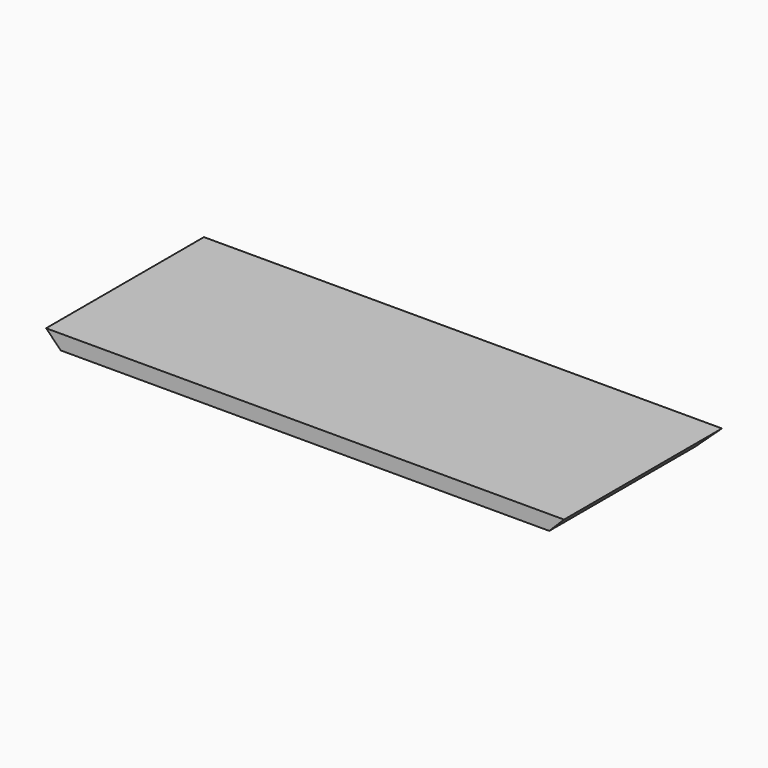
from build123d import *

# Parameters (mm, degrees)
F1_DEPTH = 254
F2_SIZE  = 19.04999


# Not quite as in the source:
# - a fillet or chamfer is up to 0.001 mm smaller than in the source, because OpenCascade refuses the exact size


with BuildPart() as f1:
    # F0 (on Front) → F1 (new body)
    with BuildSketch(Plane.XZ):
        Polygon((333.375, 9.525), (-333.375, 9.525), (-314.325, -9.525), (314.325, -9.525), align=None)
    extrude(amount=-F1_DEPTH)

    # F2 (size 19.05 in the source; OpenCascade refuses exactly that, so slightly less here)
    f2_edges = [f1.edges().sort_by_distance(p)[0] for p in [
        (0, 254, -9.525),
    ]]
    chamfer(f2_edges, length=F2_SIZE)


solid = f1.part
